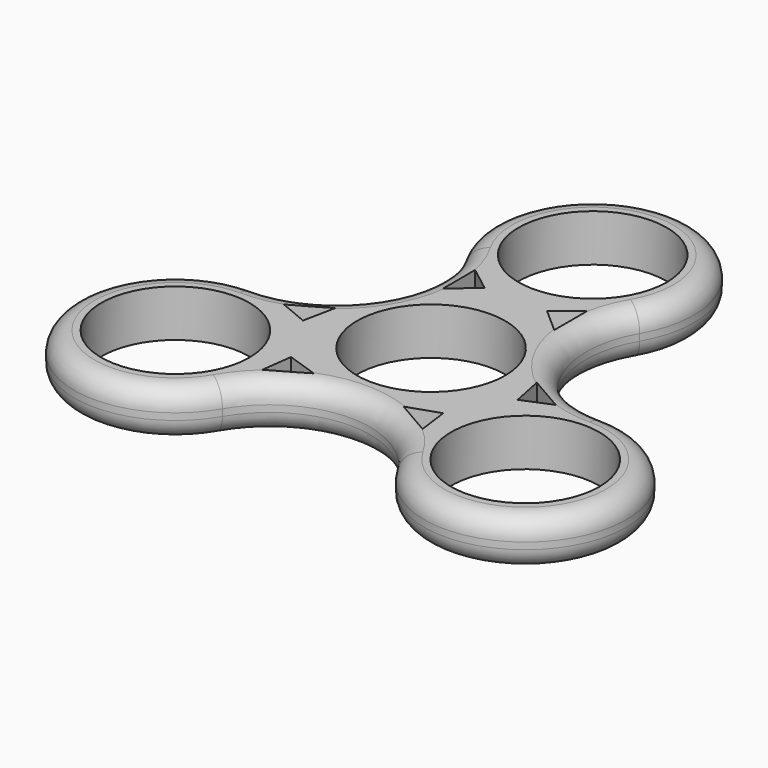
from build123d import *

# Parameters (mm, degrees)
F0_R         = 11
F1_DEPTH     = 7
F2_T2_ANGLE  = 120
F2_T4_ANGLE  = 240
F2_T6_ANGLE  = 120
F2_T8_ANGLE  = 120
F2_T10_ANGLE = 240
F2_T12_ANGLE = 120
F2_T14_ANGLE = 240
F2_T16_ANGLE = 240
F2_T18_ANGLE = 120
F2_T20_ANGLE = 240
F2_T22_ANGLE = 120
F2_T24_ANGLE = 240


# Not quite as in the source:
# - a fillet or chamfer that OpenCascade refuses, or shapes differently, is made with other operations: its cross-section is extruded or revolved along the edge and cut away or added


with BuildPart() as f1:
    # F0 (on Top) → F1 (new body)
    with BuildSketch(Plane.XY):
        with BuildLine():
            ThreePointArc((25.9807621135, 0), (12.9903810568, 7.5), (12.9903810568, 22.5))
            ThreePointArc((12.9903810568, 22.5), (0, 45), (-12.9903810568, 22.5))
            ThreePointArc((-12.9903810568, 22.5), (-12.9903810568, 7.5), (-25.9807621135, 0))
            ThreePointArc((-25.9807621135, 0), (-38.9711431703, -22.5), (-12.9903810568, -22.5))
            ThreePointArc((-12.9903810568, -22.5), (0, -15), (12.9903810568, -22.5))
            ThreePointArc((12.9903810568, -22.5), (38.9711431703, -22.5), (25.9807621135, 0))
        make_face()
        with Locations((-25.9807621135, -15)):
            Circle(F0_R, mode=Mode.SUBTRACT)
        Polygon((-11.9048568753, -16.4538883806), (-11.3039139792, -11.8745555474), (-6.6782863332, -13.4313250148), align=None, mode=Mode.SUBTRACT)
        Polygon((-14.9710118359, 0.9320968891), (-15.9356237523, -3.8521988945), (-20.2019137663, -2.0829642921), align=None, mode=Mode.SUBTRACT)
        Polygon((6.6782863332, -13.4313250148), (11.3039139792, -11.8745555474), (11.9048568753, -16.4538883806), align=None, mode=Mode.SUBTRACT)
        with Locations((25.9807621135, -15)):
            Circle(F0_R, mode=Mode.SUBTRACT)
        Circle(F0_R, mode=Mode.SUBTRACT)
        Polygon((15.9356237523, -3.8521988945), (14.9710118359, 0.9320968891), (20.2019137663, -2.0829642921), align=None, mode=Mode.SUBTRACT)
        Polygon((-8.2927255027, 12.4992281257), (-8.297056891, 18.5368526727), (-4.6317097731, 15.7267544419), align=None, mode=Mode.SUBTRACT)
        Polygon((4.6317097731, 15.7267544419), (8.297056891, 18.5368526727), (8.2927255027, 12.4992281257), align=None, mode=Mode.SUBTRACT)
        with Locations((0, 30)):
            Circle(F0_R, mode=Mode.SUBTRACT)
    extrude(amount=F1_DEPTH)

    # F2: fillet of radius 3 on 12 edges, made by hand

    # F2_s1 → F2_t2 (revolve, cut)
    with BuildSketch(Plane(origin=(-12.9903810568, 22.5, 0), x_dir=(0, 0, 1), z_dir=(-0.5, 0.8660254038, 0))):
        with BuildLine():
            ThreePointArc((4, 0), (6.1213203436, 0.8786796564), (7, 3))
            Line((7, 3), (7, 0))
            Line((7, 0), (4, 0))
        make_face()
    revolve(axis=Axis((-25.9807621135, 15, 7), (0, 0, -1)), revolution_arc=F2_T2_ANGLE, mode=Mode.SUBTRACT)

    # F2_s3 → F2_t4 (revolve, cut)
    with BuildSketch(Plane(origin=(12.9903810568, 22.5, 0), x_dir=(0, 0, 1), z_dir=(-0.5, -0.8660254038, 0))):
        with BuildLine():
            ThreePointArc((4, 0), (6.1213203436, 0.8786796564), (7, 3))
            Line((7, 3), (7, 0))
            Line((7, 0), (4, 0))
        make_face()
    revolve(axis=Axis((0, 30, 7), (0, 0, 1)), revolution_arc=F2_T4_ANGLE, mode=Mode.SUBTRACT)

    # F2_s5 → F2_t6 (revolve, cut)
    with BuildSketch(Plane.YZ.offset(25.9807621135)):
        with BuildLine():
            ThreePointArc((0, 3), (-0.8786796564, 0.8786796564), (-3, 0))
            Line((-3, 0), (0, 0))
            Line((0, 0), (0, 3))
        make_face()
    revolve(axis=Axis((25.9807621135, 15, 0), (0, 0, -1)), revolution_arc=F2_T6_ANGLE, mode=Mode.SUBTRACT)

    # F2_s7 → F2_t8 (revolve, cut)
    with BuildSketch(Plane.YZ.offset(25.9807621135)):
        with BuildLine():
            ThreePointArc((0, 4), (-0.8786796564, 6.1213203436), (-3, 7))
            Line((-3, 7), (0, 7))
            Line((0, 7), (0, 4))
        make_face()
    revolve(axis=Axis((25.9807621135, 15, 7), (0, 0, -1)), revolution_arc=F2_T8_ANGLE, mode=Mode.SUBTRACT)

    # F2_s9 → F2_t10 (revolve, cut)
    with BuildSketch(Plane(origin=(12.9903810568, -22.5, 0), x_dir=(0, 0, 1), z_dir=(-0.5, 0.8660254038, 0))):
        with BuildLine():
            ThreePointArc((4, 0), (6.1213203436, 0.8786796564), (7, 3))
            Line((7, 3), (7, 0))
            Line((7, 0), (4, 0))
        make_face()
    revolve(axis=Axis((25.9807621135, -15, 7), (0, 0, 1)), revolution_arc=F2_T10_ANGLE, mode=Mode.SUBTRACT)

    # F2_s11 → F2_t12 (revolve, cut)
    with BuildSketch(Plane(origin=(-12.9903810568, -22.5, 0), x_dir=(0, 0, 1), z_dir=(-0.5, -0.8660254038, 0))):
        with BuildLine():
            ThreePointArc((4, 0), (6.1213203436, 0.8786796564), (7, 3))
            Line((7, 3), (7, 0))
            Line((7, 0), (4, 0))
        make_face()
    revolve(axis=Axis((0, -30, 7), (0, 0, -1)), revolution_arc=F2_T12_ANGLE, mode=Mode.SUBTRACT)

    # F2_s13 → F2_t14 (revolve, cut)
    with BuildSketch(Plane.YZ.offset(-25.9807621135)):
        with BuildLine():
            ThreePointArc((0, 4), (-0.8786796564, 6.1213203436), (-3, 7))
            Line((-3, 7), (0, 7))
            Line((0, 7), (0, 4))
        make_face()
    revolve(axis=Axis((-25.9807621135, -15, 7), (0, 0, 1)), revolution_arc=F2_T14_ANGLE, mode=Mode.SUBTRACT)

    # F2_s15 → F2_t16 (revolve, cut)
    with BuildSketch(Plane(origin=(12.9903810568, 22.5, 0), x_dir=(0, 0, 1), z_dir=(-0.5, -0.8660254038, 0))):
        with BuildLine():
            ThreePointArc((3, 0), (0.8786796564, 0.8786796564), (0, 3))
            Line((0, 3), (0, 0))
            Line((0, 0), (3, 0))
        make_face()
    revolve(axis=Axis((0, 30, 0), (0, 0, 1)), revolution_arc=F2_T16_ANGLE, mode=Mode.SUBTRACT)

    # F2_s17 → F2_t18 (revolve, cut)
    with BuildSketch(Plane(origin=(-12.9903810568, 22.5, 0), x_dir=(0, 0, 1), z_dir=(-0.5, 0.8660254038, 0))):
        with BuildLine():
            ThreePointArc((3, 0), (0.8786796564, 0.8786796564), (0, 3))
            Line((0, 3), (0, 0))
            Line((0, 0), (3, 0))
        make_face()
    revolve(axis=Axis((-25.9807621135, 15, 0), (0, 0, -1)), revolution_arc=F2_T18_ANGLE, mode=Mode.SUBTRACT)

    # F2_s19 → F2_t20 (revolve, cut)
    with BuildSketch(Plane.YZ.offset(-25.9807621135)):
        with BuildLine():
            ThreePointArc((0, 3), (-0.8786796564, 0.8786796564), (-3, 0))
            Line((-3, 0), (0, 0))
            Line((0, 0), (0, 3))
        make_face()
    revolve(axis=Axis((-25.9807621135, -15, 0), (0, 0, 1)), revolution_arc=F2_T20_ANGLE, mode=Mode.SUBTRACT)

    # F2_s21 → F2_t22 (revolve, cut)
    with BuildSketch(Plane(origin=(-12.9903810568, -22.5, 0), x_dir=(0, 0, 1), z_dir=(-0.5, -0.8660254038, 0))):
        with BuildLine():
            ThreePointArc((3, 0), (0.8786796564, 0.8786796564), (0, 3))
            Line((0, 3), (0, 0))
            Line((0, 0), (3, 0))
        make_face()
    revolve(axis=Axis((0, -30, 0), (0, 0, -1)), revolution_arc=F2_T22_ANGLE, mode=Mode.SUBTRACT)

    # F2_s23 → F2_t24 (revolve, cut)
    with BuildSketch(Plane(origin=(12.9903810568, -22.5, 0), x_dir=(0, 0, 1), z_dir=(-0.5, 0.8660254038, 0))):
        with BuildLine():
            ThreePointArc((3, 0), (0.8786796564, 0.8786796564), (0, 3))
            Line((0, 3), (0, 0))
            Line((0, 0), (3, 0))
        make_face()
    revolve(axis=Axis((25.9807621135, -15, 0), (0, 0, 1)), revolution_arc=F2_T24_ANGLE, mode=Mode.SUBTRACT)


solid = f1.part
